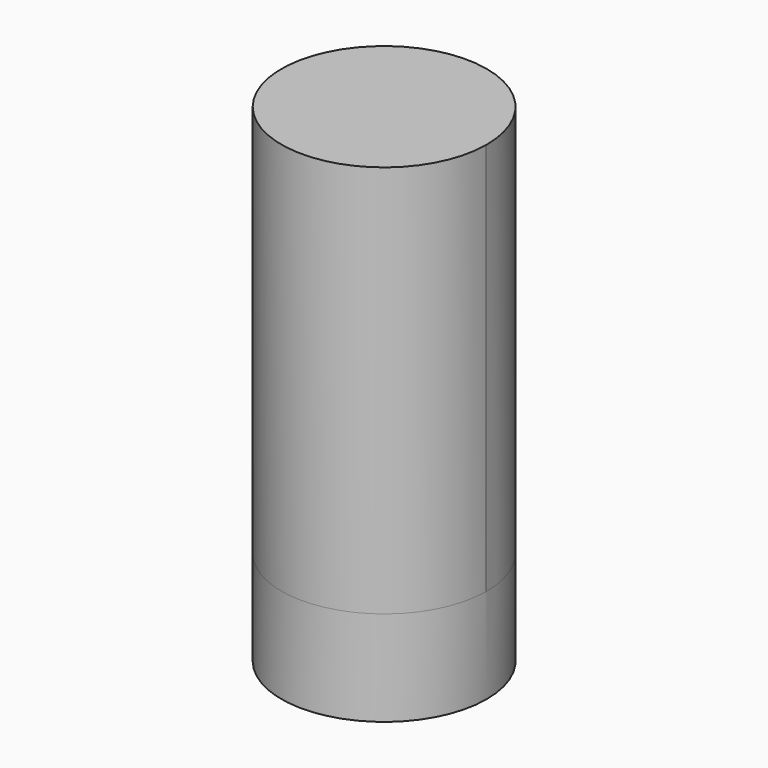
from build123d import *
from build123d import SkipClean  # not in build123d's __all__

# Parameters (mm, degrees)
F2_R     = 74.288364797
F4_DEPTH = 68.8106641173
F5_DEPTH = 284.5966219902


with BuildPart() as f4:
    # F2 (on Top) → F4 (new body)
    with BuildSketch(Plane.XY):
        with Locations((0.3392315994, 1.0795374401)):
            Circle(F2_R)
    extrude(amount=-F4_DEPTH)

    # F3 (on face) → F5 (join)
    with BuildSketch(Plane.XY):
        with BuildLine():
            Line((0, -73.2080528165), (0, 0))
            Line((0, 0), (-0.1704884926, 0))
            Line((-0.1704884926, 0), (-73.9412890176, 0))
            ThreePointArc((-73.9412890176, 0), (-51.9281732004, -51.7113665085), (0, -73.2080528165))
        make_face()
        with BuildLine():
            Line((-0.1704884926, 0), (0, 0))
            Line((0, 0), (74.6197522163, 0))
            ThreePointArc((74.6197522163, 0), (74.6256353254, 0.5397544708), (74.6275963963, 1.0795374401))
            ThreePointArc((74.6275963963, 1.0795374401), (-0.2005513699, 75.3659411662), (-73.9412890176, 0))
            Line((-73.9412890176, 0), (-0.1704884926, 0))
        make_face()
        with BuildLine():
            Line((74.6197522163, 0), (0, 0))
            Line((0, 0), (0, -73.2080528165))
            ThreePointArc((0, -73.2080528165), (52.3650262083, -51.9494908323), (74.6197522163, 0))
        make_face()
    with SkipClean():  # cleaning this boolean's faces spoils the solid; the shape is the same uncleaned
        extrude(amount=F5_DEPTH)


solid = f4.part
